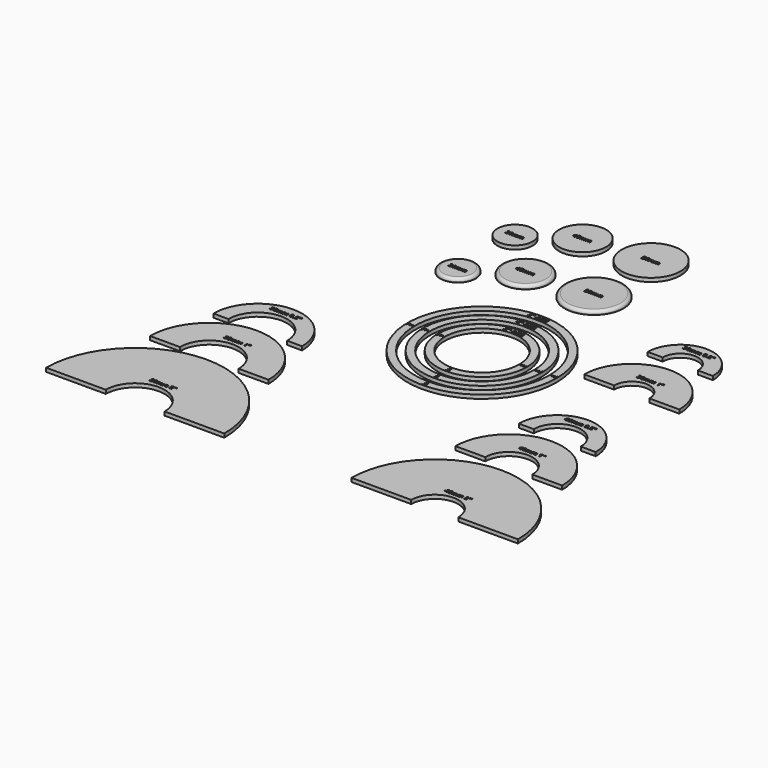
from build123d import *

# Parameters (mm, degrees)
F0_R           = 38.1
F0_R_2         = 31.75
F1_DEPTH       = 3.175
F0_R_3         = 50.8
F0_R_4         = 44.45
F0_R_5         = 63.5
F0_R_6         = 57.15
F0_R_7         = 24.99995
F0_R_8         = 19.99996
F0_R_9         = 14.99997
F2_DEPTH       = 3.175
F3_DEPTH       = 3.175
F6_TEXT_SIZE   = 4.9832272858
F6_TEXT_SIZE_2 = 4.9832330556
F6_TEXT_SIZE_3 = 4.9829861111
F7_DEPTH       = 0.79375
F9_R           = 2.54
F9_2_R         = 2.54
F9_3_R         = 2.54


# Not quite as in the source:
# - Text() gives the source's letters only with a copy of the font that has no kerning and outlines rounded to 1/6400 em; it was checked with that copy


with BuildPart() as f1:
    # F0 (on Top) → F1 (new body)
    with BuildSketch(Plane.XY):
        Circle(F0_R)
        Circle(F0_R_2, mode=Mode.SUBTRACT)
    extrude(amount=F1_DEPTH)


with BuildPart() as f1b:
    # F0 (on Top) → F1, piece 2 (new body)
    with BuildSketch(Plane.XY):
        Circle(F0_R_3)
        Circle(F0_R_4, mode=Mode.SUBTRACT)
    extrude(amount=F1_DEPTH)


with BuildPart() as f1c:
    # F0 (on Top) → F1, piece 3 (new body)
    with BuildSketch(Plane.XY):
        with BuildLine():
            Line((129.8462889602, 67.2051757574), (142.5462889602, 67.2051757574))
            ThreePointArc((142.5462889602, 67.2051757574), (114.8463189602, 94.9051457574), (87.1463489602, 67.2051757574))
            Line((87.1463489602, 67.2051757574), (99.8463489602, 67.2051757574))
            ThreePointArc((99.8463489602, 67.2051757574), (114.8463189602, 82.2051457574), (129.8462889602, 67.2051757574))
        make_face()
    extrude(amount=F1_DEPTH)


with BuildPart() as f1d:
    # F0 (on Top) → F1, piece 4 (new body)
    with BuildSketch(Plane.XY):
        with BuildLine():
            Line((137.4631165809, -66.840072607), (150.1631165809, -66.840072607))
            ThreePointArc((150.1631165809, -66.840072607), (117.4631565809, -34.140112607), (84.7631965809, -66.840072607))
            Line((84.7631965809, -66.840072607), (97.4631965809, -66.840072607))
            ThreePointArc((97.4631965809, -66.840072607), (117.4631565809, -46.840112607), (137.4631165809, -66.840072607))
        make_face()
    extrude(amount=F1_DEPTH)


with BuildPart() as f1e:
    # F0 (on Top) → F1, piece 5 (new body)
    with BuildSketch(Plane.XY):
        with BuildLine():
            Line((-109.9400649756, -69.8515027761), (-97.2400649756, -69.8515027761))
            ThreePointArc((-97.2400649756, -69.8515027761), (-134.9400149756, -32.1515527761), (-172.6399649756, -69.8515027761))
            Line((-172.6399649756, -69.8515027761), (-159.9399649756, -69.8515027761))
            ThreePointArc((-159.9399649756, -69.8515027761), (-134.9400149756, -44.8515527761), (-109.9400649756, -69.8515027761))
        make_face()
    extrude(amount=F1_DEPTH)


with BuildPart() as f1f:
    # F0 (on Top) → F1, piece 6 (new body)
    with BuildSketch(Plane.XY):
        Circle(F0_R_5)
        Circle(F0_R_6, mode=Mode.SUBTRACT)
    extrude(amount=F1_DEPTH)


with BuildPart() as f1g:
    # F0 (on Top) → F1, piece 7 (new body)
    with BuildSketch(Plane.XY):
        with Locations((6.7475424148, 110.6249988079)):
            Circle(F0_R_7)
    extrude(amount=F1_DEPTH)


with BuildPart() as f1h:
    # F0 (on Top) → F1, piece 8 (new body)
    with BuildSketch(Plane.XY):
        with Locations((-48.6690104008, 107.0450767875)):
            Circle(F0_R_8)
    extrude(amount=F1_DEPTH)


with BuildPart() as f1i:
    # F0 (on Top) → F1, piece 9 (new body)
    with BuildSketch(Plane.XY):
        with Locations((-86.7143124342, 82.7770978212)):
            Circle(F0_R_9)
    extrude(amount=F1_DEPTH)


with BuildPart() as f2:
    # F0 (on Top) → F2 (new body)
    with BuildSketch(Plane.XY):
        with BuildLine():
            Line((-109.9400649756, -69.8515027761), (-97.2400649756, -69.8515027761))
            ThreePointArc((-97.2400649756, -69.8515027761), (-134.9400149756, -32.1515527761), (-172.6399649756, -69.8515027761))
            Line((-172.6399649756, -69.8515027761), (-159.9399649756, -69.8515027761))
            ThreePointArc((-159.9399649756, -69.8515027761), (-134.9400149756, -44.8515527761), (-109.9400649756, -69.8515027761))
        make_face()
        with BuildLine():
            ThreePointArc((-172.6399649756, -69.8515027761), (-134.9400149756, -32.1515527761), (-97.2400649756, -69.8515027761))
            Line((-97.2400649756, -69.8515027761), (-84.5400649756, -69.8515027761))
            ThreePointArc((-84.5400649756, -69.8515027761), (-134.9400149756, -19.4515527761), (-185.3399649756, -69.8515027761))
            Line((-185.3399649756, -69.8515027761), (-172.6399649756, -69.8515027761))
        make_face()
    extrude(amount=F2_DEPTH)


with BuildPart() as f2b:
    # F0 (on Top) → F2, piece 2 (new body)
    with BuildSketch(Plane.XY):
        with BuildLine():
            Line((137.4631165809, -66.840072607), (150.1631165809, -66.840072607))
            ThreePointArc((150.1631165809, -66.840072607), (117.4631565809, -34.140112607), (84.7631965809, -66.840072607))
            Line((84.7631965809, -66.840072607), (97.4631965809, -66.840072607))
            ThreePointArc((97.4631965809, -66.840072607), (117.4631565809, -46.840112607), (137.4631165809, -66.840072607))
        make_face()
        with BuildLine():
            ThreePointArc((84.7631965809, -66.840072607), (117.4631565809, -34.140112607), (150.1631165809, -66.840072607))
            Line((150.1631165809, -66.840072607), (162.8631165809, -66.840072607))
            ThreePointArc((162.8631165809, -66.840072607), (117.4631565809, -21.440112607), (72.0631965809, -66.840072607))
            Line((72.0631965809, -66.840072607), (84.7631965809, -66.840072607))
        make_face()
    extrude(amount=F2_DEPTH)


with BuildPart() as f2c:
    # F0 (on Top) → F2, piece 3 (new body)
    with BuildSketch(Plane.XY):
        with BuildLine():
            Line((129.8462889602, 67.2051757574), (142.5462889602, 67.2051757574))
            ThreePointArc((142.5462889602, 67.2051757574), (114.8463189602, 94.9051457574), (87.1463489602, 67.2051757574))
            Line((87.1463489602, 67.2051757574), (99.8463489602, 67.2051757574))
            ThreePointArc((99.8463489602, 67.2051757574), (114.8463189602, 82.2051457574), (129.8462889602, 67.2051757574))
        make_face()
        with BuildLine():
            ThreePointArc((87.1463489602, 67.2051757574), (114.8463189602, 94.9051457574), (142.5462889602, 67.2051757574))
            Line((142.5462889602, 67.2051757574), (155.2462889602, 67.2051757574))
            ThreePointArc((155.2462889602, 67.2051757574), (114.8463189602, 107.6051457574), (74.4463489602, 67.2051757574))
            Line((74.4463489602, 67.2051757574), (87.1463489602, 67.2051757574))
        make_face()
    extrude(amount=F2_DEPTH)


with BuildPart() as f3:
    # F0 (on Top) → F3 (new body)
    with BuildSketch(Plane.XY):
        with BuildLine():
            Line((137.4631165809, -66.840072607), (150.1631165809, -66.840072607))
            ThreePointArc((150.1631165809, -66.840072607), (117.4631565809, -34.140112607), (84.7631965809, -66.840072607))
            Line((84.7631965809, -66.840072607), (97.4631965809, -66.840072607))
            ThreePointArc((97.4631965809, -66.840072607), (117.4631565809, -46.840112607), (137.4631165809, -66.840072607))
        make_face()
        with BuildLine():
            ThreePointArc((84.7631965809, -66.840072607), (117.4631565809, -34.140112607), (150.1631165809, -66.840072607))
            Line((150.1631165809, -66.840072607), (162.8631165809, -66.840072607))
            ThreePointArc((162.8631165809, -66.840072607), (117.4631565809, -21.440112607), (72.0631965809, -66.840072607))
            Line((72.0631965809, -66.840072607), (84.7631965809, -66.840072607))
        make_face()
        with BuildLine():
            ThreePointArc((72.0631965809, -66.840072607), (117.4631565809, -21.440112607), (162.8631165809, -66.840072607))
            Line((162.8631165809, -66.840072607), (188.2631165809, -66.840072607))
            ThreePointArc((188.2631165809, -66.840072607), (117.4631565809, 3.959887393), (46.6631965809, -66.840072607))
            Line((46.6631965809, -66.840072607), (72.0631965809, -66.840072607))
        make_face()
    extrude(amount=F3_DEPTH)


with BuildPart() as f3b:
    # F0 (on Top) → F3, piece 2 (new body)
    with BuildSketch(Plane.XY):
        with BuildLine():
            Line((-109.9400649756, -69.8515027761), (-97.2400649756, -69.8515027761))
            ThreePointArc((-97.2400649756, -69.8515027761), (-134.9400149756, -32.1515527761), (-172.6399649756, -69.8515027761))
            Line((-172.6399649756, -69.8515027761), (-159.9399649756, -69.8515027761))
            ThreePointArc((-159.9399649756, -69.8515027761), (-134.9400149756, -44.8515527761), (-109.9400649756, -69.8515027761))
        make_face()
        with BuildLine():
            ThreePointArc((-172.6399649756, -69.8515027761), (-134.9400149756, -32.1515527761), (-97.2400649756, -69.8515027761))
            Line((-97.2400649756, -69.8515027761), (-84.5400649756, -69.8515027761))
            ThreePointArc((-84.5400649756, -69.8515027761), (-134.9400149756, -19.4515527761), (-185.3399649756, -69.8515027761))
            Line((-185.3399649756, -69.8515027761), (-172.6399649756, -69.8515027761))
        make_face()
        with BuildLine():
            ThreePointArc((-185.3399649756, -69.8515027761), (-134.9400149756, -19.4515527761), (-84.5400649756, -69.8515027761))
            Line((-84.5400649756, -69.8515027761), (-59.1400649756, -69.8515027761))
            ThreePointArc((-59.1400649756, -69.8515027761), (-134.9400149756, 5.9484472239), (-210.7399649756, -69.8515027761))
            Line((-210.7399649756, -69.8515027761), (-185.3399649756, -69.8515027761))
        make_face()
    extrude(amount=F3_DEPTH)


with BuildPart() as f2b_1:
    # F4: moved
    add(f2b.part.moved(Location((0, -51.562, 0))))


with BuildPart() as f2_1:
    # F4: moved
    add(f2.part.moved(Location((0, -51.562, 0))))


with BuildPart() as f2c_1:
    # F4: moved
    add(f2c.part.moved(Location((0, -51.562, 0))))


with BuildPart() as f3_1:
    # F5: moved
    add(f3.part.moved(Location((0, -130.302, 0))))


with BuildPart() as f3b_1:
    # F5: moved
    add(f3b.part.moved(Location((0, -130.302, 0))))


with BuildPart() as f7_tool:
    # F6 (on face) → F7 (new body)
    with BuildSketch(Plane.XY.offset(3.175)):
        Polygon((50.2326415739, -1.7846057373), (50.2326415739, 0), (50.2326415739, 1.7846057373), (49.8101501593, 1.7846057373), (49.8101501593, 0), (49.8101501593, -1.7846057373), align=None)
        Polygon((47.7600015644, -1.336412057), (49.5065152239, 0), (47.7600015644, 1.336412057), (47.7600015644, 0.6682060285), (47.7600015644, 0), (47.7600015644, -0.6682060285), align=None)
        Polygon((45.616724654, -0.6682060285), (47.7600015644, -0.6682060285), (47.7600015644, 0), (47.7600015644, 0.6682060285), (45.616724654, 0.6682060285), align=None)
        Polygon((37.5457317332, -1.7845911205), (37.5385088448, 0), (37.5312940101, 1.7826012619), (37.1088187896, 1.7863003761), (37.1160174302, 0), (37.1232437756, -1.7863002643), align=None)
        Polygon((35.0715392013, -1.336412057), (36.8072816039, 0), (35.0607679444, 1.336412057), (35.0634607586, 0.6682060285), (35.0661535729, 0), (35.0688463871, -0.6682060285), align=None)
        Polygon((32.9252281568, -0.67684463), (35.0688463871, -0.6682060285), (35.0661535729, 0), (35.0634607586, 0.6682060285), (32.9198425283, 0.6595674269), align=None)
        Polygon((0.659567427, -32.9198425284), (-0.67684463, -32.9252281568), (-0.6682060284, -35.0688463871), (0, -35.0661535729), (0.6682060285, -35.0634607587), align=None)
        Polygon((0, -35.0661535729), (-0.6682060284, -35.0688463871), (-1.3364120569, -35.0715392013), (0, -36.8072816039), (1.336412057, -35.0607679444), (0.6682060285, -35.0634607587), align=None)
        Polygon((-0.6682060284, -47.7600015644), (0, -47.7600015644), (0.6682060285, -47.7600015644), (0.6682060285, -45.616724654), (-0.6682060284, -45.616724654), align=None)
        Polygon((0.6682060285, -47.7600015644), (0, -47.7600015644), (-0.6682060284, -47.7600015644), (-1.3364120569, -47.7600015644), (0, -49.5065152239), (1.336412057, -47.7600015644), align=None)
        Polygon((0, -49.8101501593), (-1.7846057372, -49.8101501593), (-1.7846057372, -50.232641574), (0, -50.2326415739), (1.7846057373, -50.2326415739), (1.7846057373, -49.8101501593), align=None)
        Polygon((-1.7863002642, -37.1232437756), (-1.7845911205, -37.5457317332), (0, -37.5385088448), (1.7826012619, -37.5312940101), (1.7863003762, -37.1088187896), (0, -37.1160174302), align=None)
        Polygon((-32.9198425283, -0.659567427), (-32.9252281567, 0.67684463), (-35.068846387, 0.6682060284), (-35.0661535728, 0), (-35.0634607586, -0.6682060285), align=None)
        Polygon((-35.0661535728, 0), (-35.068846387, 0.6682060284), (-35.0715392013, 1.3364120569), (-36.8072816039, 0), (-35.0607679444, -1.336412057), (-35.0634607586, -0.6682060285), align=None)
        Polygon((-47.7600015643, 0.6682060284), (-47.7600015643, 0), (-47.7600015643, -0.6682060285), (-45.6167246539, -0.6682060285), (-45.6167246539, 0.6682060284), align=None)
        Polygon((-47.7600015643, -0.6682060285), (-47.7600015643, 0), (-47.7600015643, 0.6682060284), (-47.7600015643, 1.3364120569), (-49.5065152238, 0), (-47.7600015643, -1.336412057), align=None)
        Polygon((-49.8101501593, 0), (-49.8101501593, 1.7846057372), (-50.2326415739, 1.7846057372), (-50.2326415739, 0), (-50.2326415739, -1.7846057373), (-49.8101501593, -1.7846057373), align=None)
        Polygon((-37.1232437756, 1.7863002642), (-37.5457317331, 1.7845911204), (-37.5385088448, 0), (-37.5312940101, -1.7826012619), (-37.1088187896, -1.7863003762), (-37.1160174302, 0), align=None)
        Polygon((62.9043756547, -1.1039322199), (62.9043756547, 0.6806735174), (62.9043756547, 2.4652792546), (62.4818842401, 2.4652792546), (62.4818842401, 0.6806735174), (62.4818842401, -1.1039322199), align=None)
        Polygon((60.4317356451, -0.6557385396), (62.1782493046, 0.6806735174), (60.4317356451, 2.0170855743), (60.4317356451, 1.3488795458), (60.4317356451, 0.6806735174), (60.4317356451, 0.0124674889), align=None)
        Polygon((58.2884587348, 0.0124674889), (60.4317356451, 0.0124674889), (60.4317356451, 0.6806735174), (60.4317356451, 1.3488795458), (58.2884587348, 1.3488795458), align=None)
        Polygon((1.3488795458, -60.4317356451), (1.3488795458, -58.2884587348), (0.0124674889, -58.2884587348), (0.0124674889, -60.4317356451), (0.6806735174, -60.4317356451), align=None)
        Polygon((2.0170855743, -60.4317356451), (1.3488795458, -60.4317356451), (0.6806735174, -60.4317356451), (0.0124674889, -60.4317356451), (-0.6557385396, -60.4317356451), (0.6806735174, -62.1782493046), align=None)
        Polygon((0.6806735174, -62.4818842401), (-1.1039322199, -62.4818842401), (-1.1039322199, -62.9043756547), (0.6806735174, -62.9043756547), (2.4652792546, -62.9043756547), (2.4652792546, -62.4818842401), align=None)
        Polygon((-60.4317356451, -1.3488795458), (-58.2884587348, -1.3488795458), (-58.2884587348, -0.0124674889), (-60.4317356451, -0.0124674889), (-60.4317356451, -0.6806735174), align=None)
        Polygon((-60.4317356451, -2.0170855743), (-60.4317356451, -1.3488795458), (-60.4317356451, -0.6806735174), (-60.4317356451, -0.0124674889), (-60.4317356451, 0.6557385396), (-62.1782493046, -0.6806735174), align=None)
        Polygon((-62.4818842401, -0.6806735174), (-62.4818842401, 1.1039322199), (-62.9043756547, 1.1039322199), (-62.9043756547, -0.6806735174), (-62.9043756547, -2.4652792546), (-62.4818842401, -2.4652792546), align=None)
        with Locations((-8.3581958281, 45.4060231895)):
            Text('4" AOE', F6_TEXT_SIZE, font='Open Sans', font_style=FontStyle.BOLD, text_align=(TextAlign.LEFT, TextAlign.BOTTOM))
        with Locations((-8.3581958281, 32.5223506988)):
            Text('3" AOE', F6_TEXT_SIZE, font='Open Sans', font_style=FontStyle.BOLD, text_align=(TextAlign.LEFT, TextAlign.BOTTOM))
        with Locations((-148.0556356031, -41.6765527761)):
            Text('50mm 0.5"', F6_TEXT_SIZE, font='Open Sans', font_style=FontStyle.BOLD, text_align=(TextAlign.LEFT, TextAlign.BOTTOM))
        with Locations((-145.9229700507, -93.2385527761)):
            Text('50mm 1"', F6_TEXT_SIZE, font='Open Sans', font_style=FontStyle.BOLD, text_align=(TextAlign.LEFT, TextAlign.BOTTOM))
        with Locations((-145.9229700507, -171.9785527761)):
            Text('50mm 2"', F6_TEXT_SIZE, font='Open Sans', font_style=FontStyle.BOLD, text_align=(TextAlign.LEFT, TextAlign.BOTTOM))
        with Locations((101.7306983326, 85.3801457574)):
            Text('30mm 0.5"', F6_TEXT_SIZE, font='Open Sans', font_style=FontStyle.BOLD, text_align=(TextAlign.LEFT, TextAlign.BOTTOM))
        with Locations((103.8633638851, 33.8181457574)):
            Text('30mm 1"', F6_TEXT_SIZE, font='Open Sans', font_style=FontStyle.BOLD, text_align=(TextAlign.LEFT, TextAlign.BOTTOM))
        with Locations((104.3475359534, -43.665112607)):
            Text('40mm 0.5"', F6_TEXT_SIZE, font='Open Sans', font_style=FontStyle.BOLD, text_align=(TextAlign.LEFT, TextAlign.BOTTOM))
        with Locations((106.4802015059, -95.227112607)):
            Text('40mm 1"', F6_TEXT_SIZE, font='Open Sans', font_style=FontStyle.BOLD, text_align=(TextAlign.LEFT, TextAlign.BOTTOM))
        with Locations((106.4802015059, -173.967112607)):
            Text('40mm 2"', F6_TEXT_SIZE, font='Open Sans', font_style=FontStyle.BOLD, text_align=(TextAlign.LEFT, TextAlign.BOTTOM))
        with Locations((-8.3582055054, 58.1060231895)):
            Text('5" AOE', F6_TEXT_SIZE_2, font='Open Sans', font_style=FontStyle.BOLD, text_align=(TextAlign.LEFT, TextAlign.BOTTOM))
        with Locations((-94.4266513285, 80.9832228212)):
            Text('30mm', F6_TEXT_SIZE_3, font='Open Sans', font_style=FontStyle.BOLD, text_align=(TextAlign.LEFT, TextAlign.BOTTOM))
        with Locations((-0.9647964795, 108.8311238079)):
            Text('50mm', F6_TEXT_SIZE_3, font='Open Sans', font_style=FontStyle.BOLD, text_align=(TextAlign.LEFT, TextAlign.BOTTOM))
        with Locations((-56.3813492951, 105.2512017875)):
            Text('40mm', F6_TEXT_SIZE_3, font='Open Sans', font_style=FontStyle.BOLD, text_align=(TextAlign.LEFT, TextAlign.BOTTOM))
    extrude(amount=-F7_DEPTH)


with BuildPart() as f1_1:
    add(f1.part)

    # F7: cut by f7_tool
    add(f7_tool.part, mode=Mode.SUBTRACT)


with BuildPart() as f1b_1:
    add(f1b.part)

    # F7: cut by f7_tool
    add(f7_tool.part, mode=Mode.SUBTRACT)


with BuildPart() as f1c_1:
    add(f1c.part)

    # F7: cut by f7_tool
    add(f7_tool.part, mode=Mode.SUBTRACT)


with BuildPart() as f1d_1:
    add(f1d.part)

    # F7: cut by f7_tool
    add(f7_tool.part, mode=Mode.SUBTRACT)


with BuildPart() as f1e_1:
    add(f1e.part)

    # F7: cut by f7_tool
    add(f7_tool.part, mode=Mode.SUBTRACT)


with BuildPart() as f1f_1:
    add(f1f.part)

    # F7: cut by f7_tool
    add(f7_tool.part, mode=Mode.SUBTRACT)


with BuildPart() as f1g_1:
    add(f1g.part)

    # F7: cut by f7_tool
    add(f7_tool.part, mode=Mode.SUBTRACT)


with BuildPart() as f1h_1:
    add(f1h.part)

    # F7: cut by f7_tool
    add(f7_tool.part, mode=Mode.SUBTRACT)


with BuildPart() as f1i_1:
    add(f1i.part)

    # F7: cut by f7_tool
    add(f7_tool.part, mode=Mode.SUBTRACT)


with BuildPart() as f2_2:
    add(f2_1.part)

    # F7: cut by f7_tool
    add(f7_tool.part, mode=Mode.SUBTRACT)


with BuildPart() as f2b_2:
    add(f2b_1.part)

    # F7: cut by f7_tool
    add(f7_tool.part, mode=Mode.SUBTRACT)


with BuildPart() as f2c_2:
    add(f2c_1.part)

    # F7: cut by f7_tool
    add(f7_tool.part, mode=Mode.SUBTRACT)


with BuildPart() as f3_2:
    add(f3_1.part)

    # F7: cut by f7_tool
    add(f7_tool.part, mode=Mode.SUBTRACT)


with BuildPart() as f3b_2:
    add(f3b_1.part)

    # F7: cut by f7_tool
    add(f7_tool.part, mode=Mode.SUBTRACT)


with BuildPart() as f8_1:
    # F8: copy of F1i
    add(f1i_1.part.moved(Location((0, 60.706, 0))))


with BuildPart() as f8_2:
    # F8: copy of F1h
    add(f1h_1.part.moved(Location((0, 60.706, 0))))


with BuildPart() as f8_3:
    # F8: copy of F1g
    add(f1g_1.part.moved(Location((0, 60.706, 0))))


with BuildPart() as f1i_2:
    add(f1i_1.part)

    # F9
    f9_edges = [f1i_2.edges().sort_by_distance(p)[0] for p in [
        (-101.714282, 82.777098, 3.175),
    ]]
    fillet(f9_edges, radius=F9_R)


with BuildPart() as f1h_2:
    add(f1h_1.part)

    # F9#2
    f9_2_edges = [f1h_2.edges().sort_by_distance(p)[0] for p in [
        (-68.66897, 107.045077, 3.175),
    ]]
    fillet(f9_2_edges, radius=F9_2_R)


with BuildPart() as f1g_2:
    add(f1g_1.part)

    # F9#3
    f9_3_edges = [f1g_2.edges().sort_by_distance(p)[0] for p in [
        (-18.252408, 110.624999, 3.175),
    ]]
    fillet(f9_3_edges, radius=F9_3_R)


solid = Compound([f1_1.part, f1b_1.part, f1c_1.part, f1d_1.part, f1e_1.part, f1f_1.part, f2_2.part, f2b_2.part, f2c_2.part, f3_2.part, f3b_2.part, f8_1.part, f8_2.part, f8_3.part, f1i_2.part, f1h_2.part, f1g_2.part])
